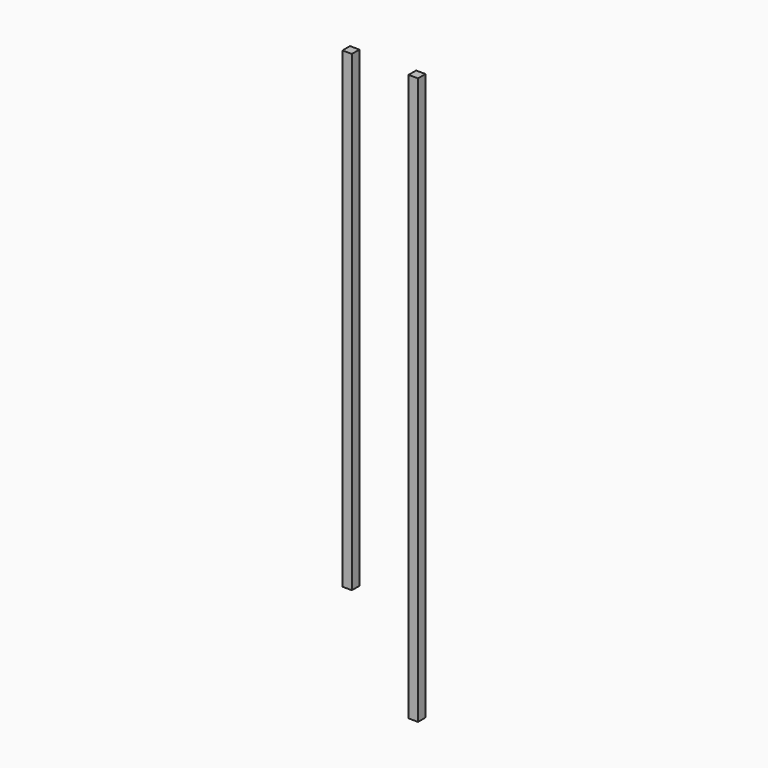
from build123d import *

# Parameters (mm, degrees)
F3_W     = 2
F3_H     = 2
F4_DEPTH = 120
F5_DEPTH = 100


# Not quite as in the source:
# - the program builds the solid bodies; features that only make, move or delete a surface that nothing else refers to are left out


with BuildPart() as f4:
    # F3 (on face) → F4 (new body)
    with BuildSketch(Plane.XY.offset(-22.2749225795)):
        with Locations((7, 0)):
            Rectangle(F3_W, F3_H)
    extrude(amount=-F4_DEPTH)


with BuildPart() as f5:
    # F3 (on face) → F5 (new body)
    with BuildSketch(Plane.XY.offset(-22.2749225795)):
        with Locations((-7, 0)):
            Rectangle(F3_W, F3_H)
    extrude(amount=-F5_DEPTH)


solid = Compound([f4.part, f5.part])
